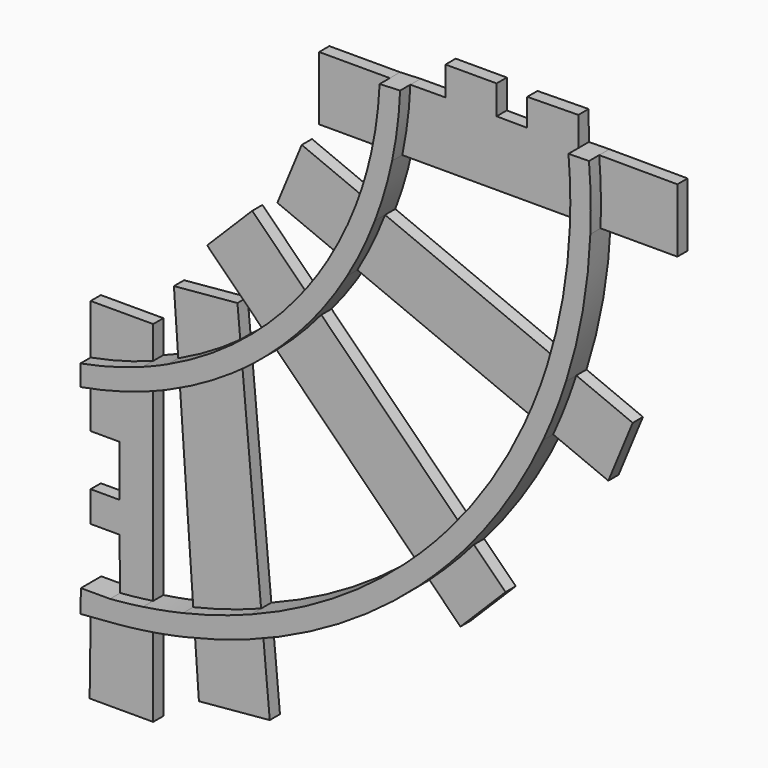
from build123d import *

# Parameters (mm, degrees)
F1_DEPTH = 3.175
F0_W     = 12.7
F0_H     = 7.1991272271
F2_DEPTH = 6.35


# Not quite as in the source:
# - a feature names something its author has since deleted; it is built from what else it names


with BuildPart() as f1:
    # F0 (on Front) → F1 (new body)
    with BuildSketch(Plane.XZ):
        with BuildLine():
            Line((0, -72.9423090816), (0, -85.3186740499))
            ThreePointArc((0, -85.3186740499), (7.8661010519, -83.5110543767), (15.5407171696, -81.0123943185))
            Line((15.5407171696, -81.0123943185), (15.5407171696, -72.9423090816))
            Line((15.5407171696, -72.9423090816), (0, -72.9423090816))
        make_face()
    extrude(amount=F1_DEPTH)


with BuildPart() as f1b:
    # F0 (on Front) → F1, piece 2 (new body)
    with BuildSketch(Plane.XZ):
        with BuildLine():
            Line((15.5407171696, -159.9892846584), (15.5407171696, -138.6477114913))
            ThreePointArc((15.5407171696, -138.6477114913), (11.6537284729, -139.1340936418), (7.7537886986, -139.5024935346))
            Line((7.7537886986, -139.5024935346), (0.0312153185, -140.1141081904))
            Line((0.0312153185, -140.1141081904), (-0.2507130796, -159.9892846584))
            Line((-0.2507130796, -159.9892846584), (15.5407171696, -159.9892846584))
        make_face()
    extrude(amount=F1_DEPTH)


with BuildPart() as f1c:
    # F0 (on Front) → F1, piece 3 (new body)
    with BuildSketch(Plane.XZ):
        with BuildLine():
            ThreePointArc((42.8434839154, -131.71122111), (34.4384994664, -134.5307535186), (25.8600517696, -136.7676624806))
            Line((25.8600517696, -136.7676624806), (26.9091483206, -151.7681628466))
            Line((26.9091483206, -151.7681628466), (44.5165795186, -150.1724443305))
            Line((44.5165795186, -150.1724443305), (42.8434839154, -131.71122111))
        make_face()
    extrude(amount=F1_DEPTH)


with BuildPart() as f1d:
    # F0 (on Front) → F1, piece 4 (new body)
    with BuildSketch(Plane.XZ):
        with BuildLine():
            Line((20.6979997025, -62.9580938124), (21.7780798158, -78.4016124462))
            ThreePointArc((21.7780798158, -78.4016124462), (29.7077533474, -74.2436885785), (37.1896057524, -69.3253618509))
            Line((37.1896057524, -69.3253618509), (36.4829087364, -61.527546032))
            Line((36.4829087364, -61.527546032), (20.6979997025, -62.9580938124))
        make_face()
    extrude(amount=F1_DEPTH)


with BuildPart() as f1e:
    # F0 (on Front) → F1, piece 5 (new body)
    with BuildSketch(Plane.XZ):
        with BuildLine():
            Line((28.9570916323, -51.3555179745), (42.6275451374, -65.0259714796))
            ThreePointArc((42.6275451374, -65.0259714796), (48.423217699, -59.6180040435), (53.7253892759, -53.7253892759))
            Line((53.7253892759, -53.7253892759), (40.1563048034, -40.1563048034))
            Line((40.1563048034, -40.1563048034), (28.9570916323, -51.3555179745))
        make_face()
    extrude(amount=F1_DEPTH)


with BuildPart() as f1f:
    # F0 (on Front) → F1, piece 6 (new body)
    with BuildSketch(Plane.XZ):
        with BuildLine():
            ThreePointArc((95.2685885997, -95.2685885997), (89.8998795149, -101.0955688623), (84.1843222901, -106.5827486323))
            Line((84.1843222901, -106.5827486323), (91.9102455753, -114.3086719175))
            Line((91.9102455753, -114.3086719175), (103.1094587464, -103.1094587464))
            Line((103.1094587464, -103.1094587464), (95.2685885997, -95.2685885997))
        make_face()
    extrude(amount=F1_DEPTH)


with BuildPart() as f1g:
    # F0 (on Front) → F1, piece 7 (new body)
    with BuildSketch(Plane.XZ):
        with BuildLine():
            ThreePointArc((120.6924286301, -49.9924408143), (118.0488124467, -57.463160193), (114.9524600656, -64.7578813318))
            Line((114.9524600656, -64.7578813318), (128.6580296336, -70.4349141269))
            Line((128.6580296336, -70.4349141269), (134.7190001265, -55.8024369617))
            Line((134.7190001265, -55.8024369617), (120.6924286301, -49.9924408143))
        make_face()
    extrude(amount=F1_DEPTH)


with BuildPart() as f1h:
    # F0 (on Front) → F1, piece 8 (new body)
    with BuildSketch(Plane.XZ):
        with BuildLine():
            Line((46.4057701695, -36.364912721), (61.5468653297, -42.6365596855))
            ThreePointArc((61.5468653297, -42.6365596856), (65.3247233264, -35.6521978828), (68.4782395176, -28.3646155356))
            Line((68.4782395176, -28.3646155356), (52.4667406624, -21.7324355559))
            Line((52.4667406624, -21.7324355559), (46.4057701695, -36.364912721))
        make_face()
    extrude(amount=F1_DEPTH)


with BuildPart() as f1i:
    # F0 (on Front) → F1, piece 9 (new body)
    with BuildSketch(Plane.XZ):
        with BuildLine():
            Line((56.7895908678, -15.8380791545), (72.2519432178, -15.8380791545))
            ThreePointArc((72.2519432178, -15.8380791545), (73.6561724133, -7.9655341121), (74.362636415, 0))
            Line((74.362636415, 0), (56.7895908678, 0))
            Line((56.7895908678, 0), (56.7895908678, -15.8380791545))
        make_face()
    extrude(amount=F1_DEPTH)


with BuildPart() as f1j:
    # F0 (on Front) → F1, piece 10 (new body)
    with BuildSketch(Plane.XZ):
        with BuildLine():
            ThreePointArc((126.3912416775, 0.0700318268), (126.8048014268, -7.8788313468), (126.7284355064, -15.8380791545))
            Line((126.7284355064, -15.8380791545), (145.8187949681, -15.8380791545))
            Line((145.8187949681, -15.8380791545), (145.8187949681, 0))
            Line((145.8187949681, 0), (126.3912416775, 0.0700318268))
        make_face()
    extrude(amount=F1_DEPTH)


with BuildPart() as f1k:
    # F0 (on Front) → F1, piece 11 (new body)
    with BuildSketch(Plane.XZ):
        with Locations((94.5389376497, 3.8679103588)):
            Rectangle(F0_W, F0_H)
        Polygon((108.5089376497, 0.2198548851), (121.2991029024, 0), (121.2089376497, 7.1882), (108.5089376497, 7.0067713694), align=None)
        with BuildLine():
            ThreePointArc((79.4563922497, 0.2198548851), (78.7929895356, -7.8514739277), (77.451129291, -15.8380791545))
            Line((77.451129291, -15.8380791545), (121.644120998, -15.8380791545))
            ThreePointArc((121.644120998, -15.8380791545), (121.724374489, -7.9135333761), (121.2991029024, 0))
            Line((121.2991029024, 0), (108.5089376497, 0.2198548851))
            Line((108.5089376497, 0.2198548851), (100.8889376497, 0.2683467453))
            Line((100.8889376497, 0.2683467453), (88.1889376497, 0.2683467453))
            Line((88.1889376497, 0.2683467453), (79.4563922497, 0.2198548851))
        make_face()
    extrude(amount=F1_DEPTH)


with BuildPart() as f1l:
    # F0 (on Front) → F1, piece 12 (new body)
    with BuildSketch(Plane.XZ):
        with BuildLine():
            ThreePointArc((15.5407171696, -86.4185788017), (7.8554934552, -88.7745728595), (0, -90.4788598418))
            Line((0, -90.4788598418), (0, -101.4183507967))
            Line((0, -101.4183507967), (7.1882, -101.4183507967))
            Line((7.1882, -101.4183507967), (7.1882, -114.1183507967))
            Line((7.1882, -114.1183507967), (0, -114.1183507967))
            Line((0, -114.1183507967), (0, -121.7383507967))
            Line((0, -121.7383507967), (7.1882, -121.7383507967))
            Line((7.1882, -121.7383507967), (7.2997089838, -134.4383507967))
            Line((7.2997089838, -134.4383507967), (7.3527172208, -134.4383507967))
            ThreePointArc((7.3527172208, -134.4383507967), (11.454370222, -134.0449461986), (15.5407171696, -133.5157079311))
            Line((15.5407171696, -133.5157079311), (15.5407171696, -86.4185788017))
        make_face()
    extrude(amount=F1_DEPTH)


with BuildPart() as f1m:
    # F0 (on Front) → F1, piece 13 (new body)
    with BuildSketch(Plane.XZ):
        with BuildLine():
            ThreePointArc((73.173293155, -30.3093704283), (70.0268183825, -37.5975502845), (66.2884926127, -44.6006060139))
            Line((66.2884926127, -44.6006060139), (110.2553632561, -62.8122801295))
            ThreePointArc((110.2553632561, -62.8122801295), (113.3544903536, -55.5182253256), (115.9821437375, -48.0413769292))
            Line((115.9821437375, -48.0413769292), (73.173293155, -30.3093704283))
        make_face()
    extrude(amount=F1_DEPTH)


with BuildPart() as f1n:
    # F0 (on Front) → F1, piece 14 (new body)
    with BuildSketch(Plane.XZ):
        with BuildLine():
            ThreePointArc((57.3333331576, -57.3333331576), (52.0152320459, -63.2104772299), (46.2300824193, -68.6285087615))
            Line((46.2300824193, -68.6285087615), (80.5873459303, -102.9857722725))
            ThreePointArc((80.5873459303, -102.9857722725), (86.3077260851, -97.50312036), (91.6668916488, -91.6668916488))
            Line((91.6668916488, -91.6668916488), (57.3333331576, -57.3333331576))
        make_face()
    extrude(amount=F1_DEPTH)


with BuildPart() as f1o:
    # F0 (on Front) → F1, piece 15 (new body)
    with BuildSketch(Plane.XZ):
        with BuildLine():
            ThreePointArc((37.719321922, -75.1703407227), (30.1382508395, -79.8486468803), (22.1558738206, -83.8034976223))
            Line((22.1558738206, -83.8034976223), (25.5013882207, -131.639314007))
            ThreePointArc((25.5013882207, -131.639314007), (34.0264897834, -129.3481143645), (42.3673240046, -126.4571911643))
            Line((42.3673240046, -126.4571911643), (37.719321922, -75.1703407227))
        make_face()
    extrude(amount=F1_DEPTH)


with BuildPart() as f2:
    # F0 (on Front) → F2 (new body)
    with BuildSketch(Plane.XZ):
        with BuildLine():
            ThreePointArc((74.362636415, 0), (73.6561724133, -7.9655341121), (72.2519432178, -15.8380791545))
            Line((72.2519432178, -15.8380791545), (77.451129291, -15.8380791545))
            ThreePointArc((77.451129291, -15.8380791545), (78.7929895356, -7.8514739277), (79.4563922497, 0.2198548851))
            Line((79.4563922497, 0.2198548851), (74.362636415, 0))
        make_face()
        with BuildLine():
            ThreePointArc((72.2519432178, -15.8380791545), (70.5908785167, -22.1693672488), (68.4782395176, -28.3646155356))
            Line((68.4782395176, -28.3646155356), (73.173293155, -30.3093704283))
            ThreePointArc((73.173293155, -30.3093704283), (75.5972198873, -23.1579757639), (77.451129291, -15.8380791545))
            Line((77.451129291, -15.8380791545), (72.2519432178, -15.8380791545))
        make_face()
        with BuildLine():
            ThreePointArc((68.4782395176, -28.3646155356), (65.3247233264, -35.6521978828), (61.5468653297, -42.6365596856))
            Line((61.5468653297, -42.6365596855), (66.2884926127, -44.6006060139))
            ThreePointArc((66.2884926127, -44.6006060139), (70.0268183825, -37.5975502845), (73.173293155, -30.3093704283))
            Line((73.173293155, -30.3093704283), (68.4782395176, -28.3646155356))
        make_face()
        with BuildLine():
            ThreePointArc((61.5468653297, -42.6365596856), (57.843462644, -48.3272179046), (53.7253892759, -53.7253892759))
            Line((53.7253892759, -53.7253892759), (57.3333331576, -57.3333331576))
            ThreePointArc((57.3333331576, -57.3333331576), (62.0696202525, -51.1489232003), (66.2884926127, -44.6006060139))
            Line((66.2884926127, -44.6006060139), (61.5468653297, -42.6365596855))
        make_face()
        with BuildLine():
            ThreePointArc((53.7253892759, -53.7253892759), (48.423217699, -59.6180040435), (42.6275451374, -65.0259714796))
            Line((42.6275451374, -65.0259714796), (46.2300824193, -68.6285087615))
            ThreePointArc((46.2300824193, -68.6285087615), (52.0152320459, -63.2104772299), (57.3333331576, -57.3333331576))
            Line((57.3333331576, -57.3333331576), (53.7253892759, -53.7253892759))
        make_face()
        with BuildLine():
            ThreePointArc((42.6275451374, -65.0259714796), (39.9496003915, -67.2275556899), (37.1896057524, -69.3253618509))
            Line((37.1896057524, -69.3253618509), (37.719321922, -75.1703407227))
            ThreePointArc((37.719321922, -75.1703407227), (42.0662817204, -72.0185674561), (46.2300824193, -68.6285087615))
            Line((46.2300824193, -68.6285087615), (42.6275451374, -65.0259714796))
        make_face()
        with BuildLine():
            ThreePointArc((37.1896057524, -69.3253618509), (29.7077533474, -74.2436885785), (21.7780798158, -78.4016124462))
            Line((21.7780798158, -78.4016124462), (22.1558738206, -83.8034976223))
            ThreePointArc((22.1558738206, -83.8034976223), (30.1382508395, -79.8486468803), (37.719321922, -75.1703407227))
            Line((37.719321922, -75.1703407227), (37.1896057524, -69.3253618509))
        make_face()
        with BuildLine():
            ThreePointArc((21.7780798158, -78.4016124462), (18.6836974569, -79.7650555136), (15.5407171696, -81.0123943185))
            Line((15.5407171696, -81.0123943185), (15.5407171696, -86.4185788017))
            ThreePointArc((15.5407171696, -86.4185788017), (18.8725439406, -85.1723775183), (22.1558738206, -83.8034976223))
            Line((22.1558738206, -83.8034976223), (21.7780798158, -78.4016124462))
        make_face()
        with BuildLine():
            ThreePointArc((15.5407171696, -81.0123943185), (7.8661010519, -83.5110543767), (0, -85.3186740499))
            Line((0, -85.3186740499), (0, -90.4788598418))
            ThreePointArc((0, -90.4788598418), (7.8554934552, -88.7745728595), (15.5407171696, -86.4185788017))
            Line((15.5407171696, -86.4185788017), (15.5407171696, -81.0123943185))
        make_face()
    extrude(amount=F2_DEPTH)


with BuildPart() as f2b:
    # F0 (on Front) → F2, piece 2 (new body)
    with BuildSketch(Plane.XZ):
        with BuildLine():
            Line((15.5407171696, -138.6477114913), (15.5407171696, -133.5157079311))
            ThreePointArc((15.5407171696, -133.5157079311), (11.454370222, -134.0449461986), (7.3527172208, -134.4383507967))
            Line((7.3527172208, -134.4383507967), (7.2997089838, -134.4383507967))
            Line((7.2997089838, -134.4383507967), (0.1117256573, -134.4383507967))
            Line((0.1117256573, -134.4383507967), (0.0312153185, -140.1141081904))
            Line((0.0312153185, -140.1141081904), (7.7537886986, -139.5024935346))
            ThreePointArc((7.7537886986, -139.5024935346), (11.6537284729, -139.1340936418), (15.5407171696, -138.6477114913))
        make_face()
        with BuildLine():
            ThreePointArc((25.5013882207, -131.639314007), (20.5402009095, -132.6791575697), (15.5407171696, -133.5157079311))
            Line((15.5407171696, -133.5157079311), (15.5407171696, -138.6477114913))
            ThreePointArc((15.5407171696, -138.6477114913), (20.7194585627, -137.8123821017), (25.8600517696, -136.7676624806))
            Line((25.8600517696, -136.7676624806), (25.5013882207, -131.639314007))
        make_face()
        with BuildLine():
            ThreePointArc((42.3673240046, -126.4571911643), (34.0264897834, -129.3481143645), (25.5013882207, -131.639314007))
            Line((25.5013882207, -131.639314007), (25.8600517696, -136.7676624806))
            ThreePointArc((25.8600517696, -136.7676624806), (34.4384994664, -134.5307535186), (42.8434839154, -131.71122111))
            Line((42.8434839154, -131.71122111), (42.3673240046, -126.4571911643))
        make_face()
        with BuildLine():
            ThreePointArc((80.5873459303, -102.9857722725), (62.5455641223, -116.4609479989), (42.3673240046, -126.4571911643))
            Line((42.3673240046, -126.4571911643), (42.8434839154, -131.71122111))
            ThreePointArc((42.8434839154, -131.71122111), (64.6997432828, -121.0979043816), (84.1843222901, -106.5827486323))
            Line((84.1843222901, -106.5827486323), (80.5873459303, -102.9857722725))
        make_face()
        with BuildLine():
            ThreePointArc((91.6668916488, -91.6668916488), (86.3077260851, -97.50312036), (80.5873459303, -102.9857722725))
            Line((80.5873459303, -102.9857722725), (84.1843222901, -106.5827486323))
            ThreePointArc((84.1843222901, -106.5827486323), (89.8998795149, -101.0955688623), (95.2685885997, -95.2685885997))
            Line((95.2685885997, -95.2685885997), (91.6668916488, -91.6668916488))
        make_face()
        with BuildLine():
            ThreePointArc((110.2553632561, -62.8122801295), (101.9626488276, -77.8847774431), (91.6668916488, -91.6668916488))
            Line((91.6668916488, -91.6668916488), (95.2685885997, -95.2685885997))
            ThreePointArc((95.2685885997, -95.2685885997), (106.1869388087, -80.7076798373), (114.9524600656, -64.7578813318))
            Line((114.9524600656, -64.7578813318), (110.2553632561, -62.8122801295))
        make_face()
        with BuildLine():
            ThreePointArc((115.9821437375, -48.0413769292), (113.3544903536, -55.5182253256), (110.2553632561, -62.8122801295))
            Line((110.2553632561, -62.8122801295), (114.9524600656, -64.7578813318))
            ThreePointArc((114.9524600656, -64.7578813318), (118.0488124467, -57.463160193), (120.6924286301, -49.9924408143))
            Line((120.6924286301, -49.9924408143), (115.9821437375, -48.0413769292))
        make_face()
        with BuildLine():
            ThreePointArc((121.644120998, -15.8380791545), (119.8774405848, -32.1268544959), (115.9821437375, -48.0413769292))
            Line((115.9821437375, -48.0413769292), (120.6924286301, -49.9924408143))
            ThreePointArc((120.6924286301, -49.9924408143), (124.8609439788, -33.1185868061), (126.7284355064, -15.8380791545))
            Line((126.7284355064, -15.8380791545), (121.644120998, -15.8380791545))
        make_face()
        with BuildLine():
            ThreePointArc((121.2991029024, 0), (121.724374489, -7.9135333761), (121.644120998, -15.8380791545))
            Line((121.644120998, -15.8380791545), (126.7284355064, -15.8380791545))
            ThreePointArc((126.7284355064, -15.8380791545), (126.8048014268, -7.8788313468), (126.3912416775, 0.0700318268))
            Line((126.3912416775, 0.0700318268), (126.3786233764, 0.0700773128))
            Line((126.3786233764, 0.0700773128), (121.2991029024, 0))
        make_face()
    extrude(amount=F2_DEPTH)


solid = Compound([f1.part, f1b.part, f1c.part, f1d.part, f1e.part, f1f.part, f1g.part, f1h.part, f1i.part, f1j.part, f1k.part, f1l.part, f1m.part, f1n.part, f1o.part, f2.part, f2b.part])
